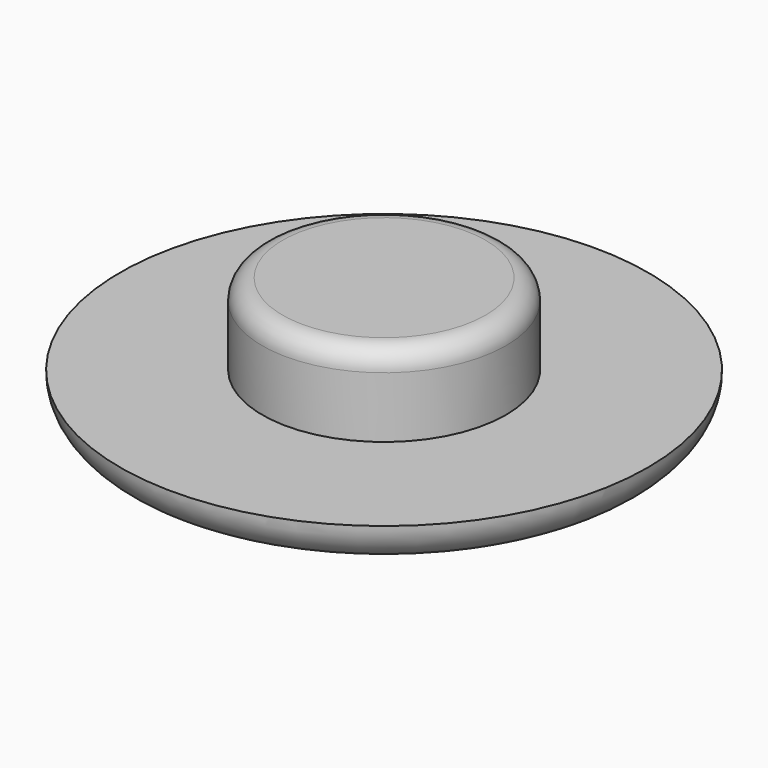
from build123d import *

# Parameters (mm, degrees)
F0_R     = 6.5
F0_R_2   = 3
F1_DEPTH = 1
F2_DEPTH = 3
F3_R     = 0.99999
F4_R     = 0.5


# Not quite as in the source:
# - a fillet or chamfer is up to 0.001 mm smaller than in the source, because OpenCascade refuses the exact size


with BuildPart() as f1:
    # F0 (on Top) → F1 (new body)
    with BuildSketch(Plane.XY):
        Circle(F0_R)
        Circle(F0_R_2, mode=Mode.SUBTRACT)
    extrude(amount=F1_DEPTH)

    # F0 (on Top) → F2 (join)
    with BuildSketch(Plane.XY):
        Circle(F0_R_2)
    extrude(amount=F2_DEPTH)

    # F3 (radius 1 in the source; OpenCascade refuses exactly that, so slightly less here)
    f3_edges = [f1.edges().sort_by_distance(p)[0] for p in [
        (-6.5, 0, 0),
    ]]
    fillet(f3_edges, radius=F3_R)

    # F4
    f4_edges = [f1.edges().sort_by_distance(p)[0] for p in [
        (-3, 0, 3),
    ]]
    fillet(f4_edges, radius=F4_R)


solid = f1.part
